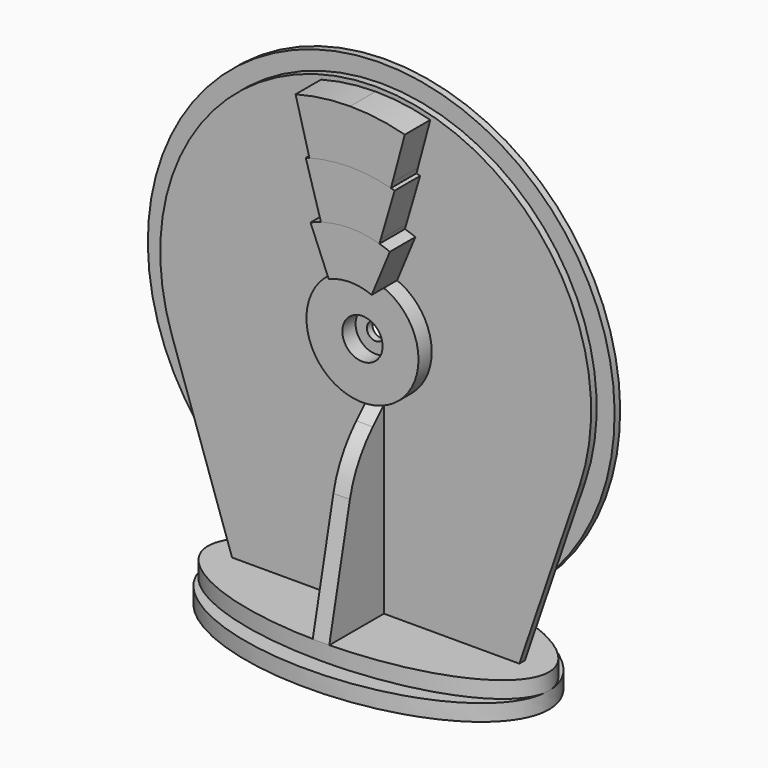
from build123d import *

# Parameters (mm, degrees)
F0_R          = 0.9525
F0_W          = 11.43
F0_H          = 37.846
F0_R_2        = 6.223
F1_DEPTH      = 2.4511
F2_R          = 39.624
F2_R_2        = 14.224
F3_DEPTH      = 11.684
F4_R          = 0.9525
F4_W          = 11.43
F4_H          = 37.846
F4_R_2        = 14.224
F5_DEPTH      = 4.9022
F7_DEPTH      = 7.3543
F7_DEPTH_BACK = 14.1361
F9_DEPTH      = 3.175
F10_R         = 0.9525
F10_W         = 11.176
F10_H         = 19.05
F10_R_2       = 2.286
F10_W_2       = 50.8
F10_H_2       = 0.254
F11_DEPTH     = 11.684
F12_W         = 50.8
F12_H         = 4.3942
F12_R         = 2.286
F12_W_2       = 13.97
F12_H_2       = 45.72
F12_R_2       = 0.9525
F13_DEPTH     = 11.684
F14_W         = 3.6322
F14_H         = 37.846
F14_W_2       = 19.05
F14_H_2       = 10.414
F15_DEPTH     = 5.842
F16_R         = 75
F18_DEPTH     = 25
F19_DEPTH     = 25


# Not quite as in the source:
# - a feature names something its author has since deleted; it is built from what else it names


with BuildPart() as f1:
    # F0 (on Front) → F1 (new body, symmetric)
    with BuildSketch(Plane.XZ):
        with BuildLine():
            Line((101.6, 22.86), (144.2136063356, 147.5732737726))
            ThreePointArc((144.2136063356, 147.5732737726), (0, 349.25), (-144.2136063356, 147.5732737726))
            Line((-144.2136063356, 147.5732737726), (-101.6, 22.86))
            Line((-101.6, 22.86), (-101.6, 2.54))
            Line((-101.6, 2.54), (-50.8, 2.54))
            Line((-50.8, 2.54), (-50.8, 22.86))
            Line((-50.8, 22.86), (0, 22.86))
            Line((0, 22.86), (50.8, 22.86))
            Line((50.8, 22.86), (50.8, 2.54))
            Line((50.8, 2.54), (101.6, 2.54))
            Line((101.6, 2.54), (101.6, 22.86))
        make_face()
        with Locations((0, 53.6575)):
            Circle(F0_R, mode=Mode.SUBTRACT)
        with Locations((0, 92.583)):
            Rectangle(F0_W, F0_H, mode=Mode.SUBTRACT)
        with Locations((0, 128.016)):
            Circle(F0_R, mode=Mode.SUBTRACT)
        with Locations((0, 196.85)):
            Circle(F0_R_2, mode=Mode.SUBTRACT)
    extrude(amount=F1_DEPTH, both=True)

    # F6 (on Front) → F7 (cut, two sides)
    with BuildSketch(Plane.XZ) as f7_sk:
        with BuildLine():
            Line((25.4, 308.6176666404), (25.4, 340.6743459919))
            ThreePointArc((25.4, 340.6743459919), (0, 342.9), (-25.4, 340.6743459919))
            Line((-25.4, 340.6743459919), (-25.4, 308.6176666404))
            ThreePointArc((-25.4, 308.6176666404), (0, 311.4675), (25.4, 308.6176666404))
        make_face()
        with BuildLine():
            Line((19.05, 270.9581999933), (19.05, 303.4283704897))
            ThreePointArc((19.05, 303.4283704897), (0, 305.1175), (-19.05, 303.4283704897))
            Line((-19.05, 303.4283704897), (-19.05, 270.9581999933))
            ThreePointArc((-19.05, 270.9581999933), (0, 273.3675), (19.05, 270.9581999933))
        make_face()
        with BuildLine():
            Line((15.24, 236.9116563094), (15.24, 265.3424846699))
            ThreePointArc((15.24, 265.3424846699), (0, 267.0175), (-15.24, 265.3424846699))
            Line((-15.24, 265.3424846699), (-15.24, 236.9116563094))
            ThreePointArc((-15.24, 236.9116563094), (0, 239.7125), (15.24, 236.9116563094))
        make_face()
    extrude(amount=-F7_DEPTH, mode=Mode.SUBTRACT)
    extrude(f7_sk.sketch, amount=F7_DEPTH_BACK, mode=Mode.SUBTRACT)


with BuildPart() as f3:
    # F2 (on face) → F3 (new body)
    with BuildSketch(Plane.XZ.offset(2.4511)):
        with Locations((0, 196.85)):
            Circle(F2_R)
        with Locations((0, 196.85)):
            Circle(F2_R_2, mode=Mode.SUBTRACT)
    extrude(amount=F3_DEPTH)


with BuildPart() as f5:
    # F4 (on face) → F5 (new body)
    with BuildSketch(Plane(origin=(0, 2.4511, 0), x_dir=(-1, 0, 0), z_dir=(0, 1, 0))):
        with BuildLine():
            ThreePointArc((123.6816370741, 87.4842711328), (154.3985885313, 138.3770501896), (165.1, 196.85))
            ThreePointArc((165.1, 196.85), (-58.4729498104, 351.2485885313), (-123.6816370741, 87.4842711328))
            Line((-123.6816370741, 87.4842711328), (-144.2136063356, 147.5732737726))
            ThreePointArc((-144.2136063356, 147.5732737726), (0, 349.25), (144.2136063356, 147.5732737726))
            Line((144.2136063356, 147.5732737726), (123.6816370741, 87.4842711328))
        make_face()
        with BuildLine():
            Line((-144.2136063356, 147.5732737726), (-123.6816370741, 87.4842711328))
            ThreePointArc((-123.6816370741, 87.4842711328), (0, 31.75), (123.6816370741, 87.4842711328))
            Line((123.6816370741, 87.4842711328), (144.2136063356, 147.5732737726))
            ThreePointArc((144.2136063356, 147.5732737726), (0, 349.25), (-144.2136063356, 147.5732737726))
        make_face()
        with Locations((0, 53.6575)):
            Circle(F4_R, mode=Mode.SUBTRACT)
        with Locations((0, 92.583)):
            Rectangle(F4_W, F4_H, mode=Mode.SUBTRACT)
        with Locations((0, 128.016)):
            Circle(F4_R, mode=Mode.SUBTRACT)
        with Locations((0, 196.85)):
            Circle(F4_R_2, mode=Mode.SUBTRACT)
        with Locations((0, 53.6575)):
            Circle(F4_R)
        with Locations((0, 92.583)):
            Rectangle(F4_W, F4_H)
        with Locations((0, 128.016)):
            Circle(F4_R)
    extrude(amount=F5_DEPTH)


with BuildPart() as f9:
    # F8 (on Front) → F9 (new body, symmetric)
    with BuildSketch(Plane.XZ):
        with BuildLine():
            ThreePointArc((-13.97, 238.7130703156), (0, 240.9825), (13.97, 238.7130703156))
            Line((13.97, 238.7130703156), (13.97, 264.3163220151))
            ThreePointArc((13.97, 264.3163220151), (0, 265.7475), (-13.97, 264.3163220151))
            Line((-13.97, 264.3163220151), (-13.97, 238.7130703156))
        make_face()
    extrude(amount=F9_DEPTH, both=True)


with BuildPart() as f9b:
    # F8 (on Front) → F9, piece 2 (new body, symmetric)
    with BuildSketch(Plane.XZ):
        with BuildLine():
            ThreePointArc((-24.13, 310.1975), (0, 312.7375), (24.13, 310.1975))
            Line((24.13, 310.1975), (24.13, 339.6050051662))
            ThreePointArc((24.13, 339.6050051662), (0, 341.63), (-24.13, 339.6050051662))
            Line((-24.13, 339.6050051662), (-24.13, 310.1975))
        make_face()
    extrude(amount=F9_DEPTH, both=True)


with BuildPart() as f9c:
    # F8 (on Front) → F9, piece 3 (new body, symmetric)
    with BuildSketch(Plane.XZ):
        with BuildLine():
            Line((17.78, 272.5782427912), (17.78, 302.3598886657))
            ThreePointArc((17.78, 302.3598886657), (0, 303.8475), (-17.78, 302.3598886657))
            Line((-17.78, 302.3598886657), (-17.78, 272.5782427912))
            ThreePointArc((-17.78, 272.5782427912), (0, 274.6375), (17.78, 272.5782427912))
        make_face()
    extrude(amount=F9_DEPTH, both=True)


with BuildPart() as f11:
    # F10 (on face) → F11 (new body)
    with BuildSketch(Plane(origin=(0, 0, 22.86), x_dir=(1, 0, 0), z_dir=(0, 0, -1))):
        with BuildLine():
            add(Edge.make_bspline(
                [(0, 50.8), (-208.9719299332, 50.8), (-104.4859649666, -25.4), (0, -101.6), (104.4859649666, -25.4), (208.9719299332, 50.8), (0, 50.8)],
                knots=[4.7123889804, 4.7123889804, 4.7123889804, 6.8067840828, 6.8067840828, 8.9011791852, 8.9011791852, 10.9955742876, 10.9955742876, 10.9955742876], degree=2, weights=[1, 0.5, 1, 0.5, 1, 0.5, 1]))
        make_face()
        Polygon((-50.8, -2.4511), (-101.6, -2.4511), (-101.6, -2.1971), (-101.6, 2.1971), (-101.6, 2.4511), (-50.8, 2.4511), (50.8, 2.4511), (101.6, 2.4511), (101.6, 2.1971), (101.6, -2.1971), (101.6, -2.4511), (50.8, -2.4511), align=None, mode=Mode.SUBTRACT)
        with Locations((0, 9.525)):
            Circle(F10_R, mode=Mode.SUBTRACT)
        with Locations((0, 25.4)):
            Rectangle(F10_W, F10_H, mode=Mode.SUBTRACT)
        with Locations((0, 40.005)):
            Circle(F10_R, mode=Mode.SUBTRACT)
        Polygon((-50.8, -2.1971), (-50.8, -2.4511), (50.8, -2.4511), (50.8, -2.1971), (50.8, 2.1971), (50.8, 2.4511), (-50.8, 2.4511), (-50.8, 2.1971), align=None)
        with Locations((-40.64, 0)):
            Circle(F10_R_2, mode=Mode.SUBTRACT)
        with Locations((40.64, 0)):
            Circle(F10_R_2, mode=Mode.SUBTRACT)
        with Locations((-76.2, -2.3241)):
            Rectangle(F10_W_2, F10_H_2)
        with Locations((-76.2, 2.3241)):
            Rectangle(F10_W_2, F10_H_2)
        with Locations((76.2, 2.3241)):
            Rectangle(F10_W_2, F10_H_2)
        with Locations((76.2, -2.3241)):
            Rectangle(F10_W_2, F10_H_2)
    extrude(amount=F11_DEPTH)


with BuildPart() as f13:
    # F12 (on face) → F13 (new body)
    with BuildSketch(Plane(origin=(0, 0, 11.176), x_dir=(1, 0, 0), z_dir=(0, 0, -1))):
        with BuildLine():
            add(Edge.make_bspline(
                [(0, 50.8), (-120.6499959128, 50.8), (-120.65, 1.7209e-06)],
                knots=[4.7123889804, 4.7123889804, 4.7123889804, 6.2455925735, 6.2455925735, 6.2455925735], degree=2, weights=[1, 0.6339746041, 0.80384757]))
            add(Edge.make_bspline(
                [(-120.65, 1.7209e-06), (-120.6500010952, -13.6118181768), (-104.4859649666, -25.4), (0, -101.6), (104.4859649666, -25.4), (120.6499986646, -13.6118199494), (120.65, -2.0984e-06)],
                knots=[6.2455925735, 6.2455925735, 6.2455925735, 6.8067840828, 6.8067840828, 8.9011791852, 8.9011791852, 9.4623706213, 9.4623706213, 9.4623706213], degree=2, weights=[0.80384757, 0.8660253959, 1, 0.5, 1, 0.8660254134, 0.8038475862]))
            add(Edge.make_bspline(
                [(120.65, -2.0984e-06), (120.6500049837, 50.8), (0, 50.8)],
                knots=[9.4623706213, 9.4623706213, 9.4623706213, 10.9955742876, 10.9955742876, 10.9955742876], degree=2, weights=[0.8038475862, 0.6339745866, 1]))
        make_face()
        with Locations((-76.2, 0)):
            Rectangle(F12_W, F12_H, mode=Mode.SUBTRACT)
        with Locations((-40.64, 0)):
            Circle(F12_R, mode=Mode.SUBTRACT)
        with Locations((40.64, 0)):
            Circle(F12_R, mode=Mode.SUBTRACT)
        with Locations((0, 22.86)):
            Rectangle(F12_W_2, F12_H_2, mode=Mode.SUBTRACT)
        with Locations((76.2, 0)):
            Rectangle(F12_W, F12_H, mode=Mode.SUBTRACT)
        with BuildLine():
            add(Edge.make_bspline(
                [(120.65, -2.0984e-06), (120.650003987, 63.5), (0, 63.5)],
                knots=[3.1415926205, 3.1415926205, 3.1415926205, 4.7123889804, 4.7123889804, 4.7123889804], degree=2, weights=[1, 0.7071067695, 1]))
            add(Edge.make_bspline(
                [(0, 63.5), (-120.6499967302, 63.5), (-120.65, 1.7209e-06)],
                knots=[4.7123889804, 4.7123889804, 4.7123889804, 6.2831852801, 6.2831852801, 6.2831852801], degree=2, weights=[1, 0.7071067908, 1]))
            add(Edge.make_bspline(
                [(0, 50.8), (-120.6499959128, 50.8), (-120.65, 1.7209e-06)],
                knots=[4.7123889804, 4.7123889804, 4.7123889804, 6.2455925735, 6.2455925735, 6.2455925735], degree=2, weights=[1, 0.6339746041, 0.80384757]))
            add(Edge.make_bspline(
                [(120.65, -2.0984e-06), (120.6500049837, 50.8), (0, 50.8)],
                knots=[9.4623706213, 9.4623706213, 9.4623706213, 10.9955742876, 10.9955742876, 10.9955742876], degree=2, weights=[0.8038475862, 0.6339745866, 1]))
        make_face()
        with BuildLine():
            add(Edge.make_bspline(
                [(-120.65, 1.7209e-06), (-120.6500010952, -13.6118181768), (-104.4859649666, -25.4), (0, -101.6), (104.4859649666, -25.4), (120.6499986646, -13.6118199494), (120.65, -2.0984e-06)],
                knots=[6.2455925735, 6.2455925735, 6.2455925735, 6.8067840828, 6.8067840828, 8.9011791852, 8.9011791852, 9.4623706213, 9.4623706213, 9.4623706213], degree=2, weights=[0.80384757, 0.8660253959, 1, 0.5, 1, 0.8660254134, 0.8038475862]))
            add(Edge.make_bspline(
                [(-120.65, 1.7209e-06), (-120.6500032698, -63.4999980903), (-3.6284e-06, -63.5), (120.649996013, -63.5000019097), (120.65, -2.0984e-06)],
                knots=[6.2831852801, 6.2831852801, 6.2831852801, 7.8539816039, 7.8539816039, 9.4247779277, 9.4247779277, 9.4247779277], degree=2, weights=[1, 0.7071067822, 1, 0.7071067822, 1]))
        make_face()
        with Locations((-40.64, 0)):
            Circle(F12_R)
        with Locations((-40.64, 0)):
            Circle(F12_R_2, mode=Mode.SUBTRACT)
        with Locations((40.64, 0)):
            Circle(F12_R)
        with Locations((40.64, 0)):
            Circle(F12_R_2, mode=Mode.SUBTRACT)
    extrude(amount=F13_DEPTH)


with BuildPart() as f15:
    # F14 (on Right) → F15 (new body, symmetric)
    with BuildSketch(Plane.YZ):
        with Locations((-0.635, 92.583)):
            Rectangle(F14_W, F14_H)
        with Locations((-25.4, 17.653)):
            Rectangle(F14_W_2, F14_H_2)
        Polygon((-15.875, 22.86), (-2.4511, 22.86), (-2.4511, 73.66), (-2.4511, 111.506), (-2.4511, 147.5732737726), (-2.4511, 153.035), (-27.8511, 127.635), (-50.8, 22.86), (-34.925, 22.86), align=None)
    extrude(amount=F15_DEPTH, both=True)

    # F16
    f16_edges = [f15.edges().sort_by_distance(p)[0] for p in [
        (0, -27.8511, 127.635),
    ]]
    fillet(f16_edges, radius=F16_R)


with BuildPart() as f18:
    # F17 (on Front) → F18 (new body)
    with BuildSketch(Plane.XZ):
        with BuildLine():
            Line((-28.0669596382, 264.6096346132), (-15.187748722, 233.5164689465))
            ThreePointArc((-15.187748722, 233.5164689465), (-13.2071426898, 234.2755131992), (-11.188813121, 234.9276590298))
            Line((-11.188813121, 234.9276590298), (-12.0839181707, 237.9738717522))
            Line((-12.0839181707, 237.9738717522), (-20.6672922558, 267.1847262192))
            Line((-20.6672922558, 267.1847262192), (-20.7881839977, 267.1847262192))
            ThreePointArc((-20.7881839977, 267.1847262192), (-24.4614807221, 265.9930276104), (-28.0669596382, 264.6096346132))
        make_face()
        with BuildLine():
            ThreePointArc((11.188813121, 234.9276590298), (13.2071426898, 234.2755131992), (15.187748722, 233.5164689465))
            Line((15.187748722, 233.5164689465), (28.0669596382, 264.6096346132))
            ThreePointArc((28.0669596382, 264.6096346132), (24.4614807221, 265.9930276104), (20.7881839977, 267.1847262192))
            Line((20.7881839977, 267.1847262192), (20.6672922558, 267.1847262192))
            Line((20.6672922558, 267.1847262192), (12.0839181707, 237.9738717522))
            Line((12.0839181707, 237.9738717522), (11.188813121, 234.9276590298))
        make_face()
        with BuildLine():
            Line((-12.0839181707, 237.9738717522), (-11.188813121, 234.9276590298))
            ThreePointArc((-11.188813121, 234.9276590298), (-10.7311195072, 235.0591707627), (-10.2718808525, 235.1851812308))
            Line((-10.2718808525, 235.1851812308), (-11.0936313207, 238.2519957293))
            ThreePointArc((-11.0936313207, 238.2519957293), (-11.5896090678, 238.1159044237), (-12.0839181707, 237.9738717522))
        make_face()
        with BuildLine():
            Line((-11.0936313207, 238.2519957293), (-10.2718808525, 235.1851812308))
            ThreePointArc((-10.2718808525, 235.1851812308), (-5.1802582537, 236.1979679358), (0, 236.5375))
            Line((0, 236.5375), (0, 239.7125))
            ThreePointArc((0, 239.7125), (-5.594678914, 239.3458053706), (-11.0936313207, 238.2519957293))
        make_face()
        with BuildLine():
            ThreePointArc((0, 236.5375), (5.1802582537, 236.1979679358), (10.2718808525, 235.1851812308))
            Line((10.2718808525, 235.1851812308), (11.0936313207, 238.2519957293))
            ThreePointArc((11.0936313207, 238.2519957293), (5.594678914, 239.3458053706), (0, 239.7125))
            Line((0, 239.7125), (0, 236.5375))
        make_face()
        with BuildLine():
            ThreePointArc((10.2718808525, 235.1851812308), (10.7311195072, 235.0591707627), (11.188813121, 234.9276590298))
            Line((11.188813121, 234.9276590298), (12.0839181707, 237.9738717522))
            ThreePointArc((12.0839181707, 237.9738717522), (11.5896090678, 238.1159044237), (11.0936313207, 238.2519957293))
            Line((11.0936313207, 238.2519957293), (10.2718808525, 235.1851812308))
        make_face()
        with BuildLine():
            ThreePointArc((11.0936313207, 238.2519957293), (11.5896090678, 238.1159044237), (12.0839181707, 237.9738717522))
            Line((12.0839181707, 237.9738717522), (20.6672922558, 267.1847262192))
            Line((20.6672922558, 267.1847262192), (18.8461330903, 267.1847262192))
            Line((18.8461330903, 267.1847262192), (11.0936313207, 238.2519957293))
        make_face()
        with BuildLine():
            ThreePointArc((0, 239.7125), (5.594678914, 239.3458053706), (11.0936313207, 238.2519957293))
            Line((11.0936313207, 238.2519957293), (18.8461330903, 267.1847262192))
            Line((18.8461330903, 267.1847262192), (0, 267.1847262192))
            Line((0, 267.1847262192), (-18.8461330903, 267.1847262192))
            Line((-18.8461330903, 267.1847262192), (-11.0936313207, 238.2519957293))
            ThreePointArc((-11.0936313207, 238.2519957293), (-5.594678914, 239.3458053706), (0, 239.7125))
        make_face()
        with BuildLine():
            Line((-20.6672922558, 267.1847262192), (-12.0839181707, 237.9738717522))
            ThreePointArc((-12.0839181707, 237.9738717522), (-11.5896090678, 238.1159044237), (-11.0936313207, 238.2519957293))
            Line((-11.0936313207, 238.2519957293), (-18.8461330903, 267.1847262192))
            Line((-18.8461330903, 267.1847262192), (-20.6672922558, 267.1847262192))
        make_face()
        with BuildLine():
            Line((-18.9824358154, 267.6934149146), (-18.8461330903, 267.1847262192))
            Line((-18.8461330903, 267.1847262192), (0, 267.1847262192))
            Line((0, 267.1847262192), (0, 270.1925))
            ThreePointArc((0, 270.1925), (-9.5731172529, 269.5650447453), (-18.9824358154, 267.6934149146))
        make_face()
        with BuildLine():
            Line((0, 267.1847262192), (18.8461330903, 267.1847262192))
            Line((18.8461330903, 267.1847262192), (18.9824358154, 267.6934149146))
            ThreePointArc((18.9824358154, 267.6934149146), (9.5731172529, 269.5650447453), (0, 270.1925))
            Line((0, 270.1925), (0, 267.1847262192))
        make_face()
        with BuildLine():
            Line((18.8461330903, 267.1847262192), (20.6672922558, 267.1847262192))
            Line((20.6672922558, 267.1847262192), (20.6769266477, 267.2175138871))
            ThreePointArc((20.6769266477, 267.2175138871), (19.8311088493, 267.4605475695), (18.9824358154, 267.6934149146))
            Line((18.9824358154, 267.6934149146), (18.8461330903, 267.1847262192))
        make_face()
        with BuildLine():
            Line((-20.6769266477, 267.2175138871), (-20.6672922558, 267.1847262192))
            Line((-20.6672922558, 267.1847262192), (-18.8461330903, 267.1847262192))
            Line((-18.8461330903, 267.1847262192), (-18.9824358154, 267.6934149146))
            ThreePointArc((-18.9824358154, 267.6934149146), (-19.8311088493, 267.4605475695), (-20.6769266477, 267.2175138871))
        make_face()
    extrude(amount=F18_DEPTH)


with BuildPart() as f18b:
    # F17 (on Front) → F18, piece 2 (new body)
    with BuildSketch(Plane.XZ):
        with BuildLine():
            Line((-29.8609278775, 308.2925), (0, 308.2925))
            Line((0, 308.2925), (29.8609278775, 308.2925))
            Line((29.8609278775, 308.2925), (38.6222720054, 340.990281428))
            ThreePointArc((38.6222720054, 340.990281428), (19.477771034, 344.7983594385), (0, 346.075))
            ThreePointArc((0, 346.075), (-19.477771034, 344.7983594385), (-38.6222720054, 340.990281428))
            Line((-38.6222720054, 340.990281428), (-29.8609278775, 308.2925))
        make_face()
        with BuildLine():
            ThreePointArc((0, 308.2925), (14.5069609881, 307.3442482175), (28.7670457554, 304.5156300068))
            Line((28.7670457554, 304.5156300068), (28.8489186129, 304.5156300068))
            Line((28.8489186129, 304.5156300068), (29.8609278775, 308.2925))
            Line((29.8609278775, 308.2925), (0, 308.2925))
        make_face()
        with BuildLine():
            Line((-28.8489186129, 304.5156300068), (-28.7670457554, 304.5156300068))
            ThreePointArc((-28.7670457554, 304.5156300068), (-14.5069609881, 307.3442482175), (0, 308.2925))
            Line((0, 308.2925), (-29.8609278775, 308.2925))
            Line((-29.8609278775, 308.2925), (-28.8489186129, 304.5156300068))
        make_face()
    extrude(amount=F18_DEPTH)


with BuildPart() as f19:
    # F17 (on Front) → F19 (new body)
    with BuildSketch(Plane.XZ):
        with BuildLine():
            Line((-31.4181872439, 303.7720665558), (-21.5511023324, 270.1925))
            Line((-21.5511023324, 270.1925), (-19.6520636459, 270.1925))
            Line((-19.6520636459, 270.1925), (-28.8434414338, 304.4951888962))
            ThreePointArc((-28.8434414338, 304.4951888962), (-30.1329835762, 304.1413515016), (-31.4181872439, 303.7720665558))
        make_face()
        with BuildLine():
            Line((-21.5511023324, 270.1925), (-20.6769266477, 267.2175138871))
            ThreePointArc((-20.6769266477, 267.2175138871), (-19.8311088493, 267.4605475695), (-18.9824358154, 267.6934149146))
            Line((-18.9824358154, 267.6934149146), (-19.6520636459, 270.1925))
            Line((-19.6520636459, 270.1925), (-21.5511023324, 270.1925))
        make_face()
        with BuildLine():
            Line((-19.6520636459, 270.1925), (-18.9824358154, 267.6934149146))
            ThreePointArc((-18.9824358154, 267.6934149146), (-9.5731172529, 269.5650447453), (0, 270.1925))
            Line((0, 270.1925), (-19.6520636459, 270.1925))
        make_face()
        with BuildLine():
            Line((-19.6520636459, 270.1925), (0, 270.1925))
            Line((0, 270.1925), (19.6520636459, 270.1925))
            Line((19.6520636459, 270.1925), (28.8434414338, 304.4951888962))
            ThreePointArc((28.8434414338, 304.4951888962), (28.8052454078, 304.5054162281), (28.7670457554, 304.5156300068))
            Line((28.7670457554, 304.5156300068), (11.4001610292, 304.5156300068))
            Line((11.4001610292, 304.5156300068), (-11.4001610292, 304.5156300068))
            Line((-11.4001610292, 304.5156300068), (-28.7670457554, 304.5156300068))
            ThreePointArc((-28.7670457554, 304.5156300068), (-28.8052454078, 304.5054162281), (-28.8434414338, 304.4951888962))
            Line((-28.8434414338, 304.4951888962), (-19.6520636459, 270.1925))
        make_face()
        with BuildLine():
            ThreePointArc((0, 270.1925), (9.5731172529, 269.5650447453), (18.9824358154, 267.6934149146))
            Line((18.9824358154, 267.6934149146), (19.6520636459, 270.1925))
            Line((19.6520636459, 270.1925), (0, 270.1925))
        make_face()
        with BuildLine():
            ThreePointArc((18.9824358154, 267.6934149146), (19.8311088493, 267.4605475695), (20.6769266477, 267.2175138871))
            Line((20.6769266477, 267.2175138871), (21.5511023324, 270.1925))
            Line((21.5511023324, 270.1925), (19.6520636459, 270.1925))
            Line((19.6520636459, 270.1925), (18.9824358154, 267.6934149146))
        make_face()
        with BuildLine():
            Line((19.6520636459, 270.1925), (21.5511023324, 270.1925))
            Line((21.5511023324, 270.1925), (31.4181872439, 303.7720665558))
            ThreePointArc((31.4181872439, 303.7720665558), (30.1329835762, 304.1413515016), (28.8434414338, 304.4951888962))
            Line((28.8434414338, 304.4951888962), (19.6520636459, 270.1925))
        make_face()
        with BuildLine():
            ThreePointArc((0, 308.2925), (-14.5069609881, 307.3442482175), (-28.7670457554, 304.5156300068))
            Line((-28.7670457554, 304.5156300068), (-11.4001610292, 304.5156300068))
            ThreePointArc((-11.4001610292, 304.5156300068), (-5.7080188984, 304.9669277981), (0, 305.1175))
            Line((0, 305.1175), (0, 308.2925))
        make_face()
        with BuildLine():
            Line((-11.4001610292, 304.5156300068), (11.4001610292, 304.5156300068))
            ThreePointArc((11.4001610292, 304.5156300068), (5.7080188984, 304.9669277981), (0, 305.1175))
            ThreePointArc((0, 305.1175), (-5.7080188984, 304.9669277981), (-11.4001610292, 304.5156300068))
        make_face()
        with BuildLine():
            Line((11.4001610292, 304.5156300068), (28.7670457554, 304.5156300068))
            ThreePointArc((28.7670457554, 304.5156300068), (14.5069609881, 307.3442482175), (0, 308.2925))
            Line((0, 308.2925), (0, 305.1175))
            ThreePointArc((0, 305.1175), (5.7080188984, 304.9669277981), (11.4001610292, 304.5156300068))
        make_face()
    extrude(amount=F19_DEPTH)


solid = Compound([f1.part, f3.part, f5.part, f9.part, f9b.part, f9c.part, f11.part, f13.part, f15.part, f18.part, f18b.part, f19.part])
